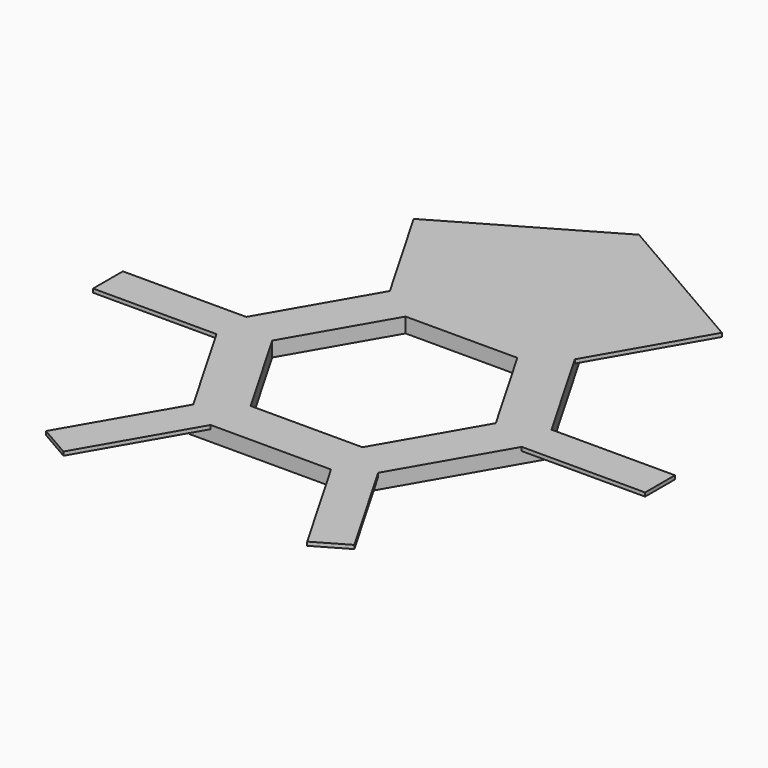
from build123d import *

# Parameters (mm, degrees)
F1_DEPTH = 152.4
F2_DEPTH = 457.2


# Not quite as in the source:
# - the program builds the solid bodies; features that only make, move or delete a surface that nothing else refers to are left out


with BuildPart() as f1:
    # F0 (on Top) → F1 (new body)
    with BuildSketch(Plane.XY):
        Polygon((6247.1608527394, 762), (6687.1017578619, 0), (6247.1608527394, -762), (11296.6448630235, -762), (11296.6448630235, 762), align=None)
        Polygon((6247.1608527394, -762), (6687.1017578619, 0), (6247.1608527394, 762), (3783.4917840535, 5029.2), (3343.550878931, 5791.2), (2463.669068686, 5791.2), (-2463.669068686, 5791.2), (-3343.550878931, 5791.2), (-3783.4917840535, 5029.2), (-6247.1608527394, 762), (-6687.1017578619, 0), (-6247.1608527394, -762), (-3783.4917840535, -5029.2), (-3343.550878931, -5791.2), (-2463.669068686, -5791.2), (2463.669068686, -5791.2), (3343.550878931, -5791.2), (3783.4917840535, -5029.2), align=None)
        Polygon((2287.692706637, 3962.4), (4575.3854132739, 0), (2287.692706637, -3962.4), (-2287.692706637, -3962.4), (-4575.3854132739, 0), (-2287.692706637, 3962.4), align=None, mode=Mode.SUBTRACT)
        Polygon((6308.2337891955, -9402.1814289093), (3783.4917840535, -5029.2), (3343.550878931, -5791.2), (2463.669068686, -5791.2), (4988.411073828, -10164.1814289093), align=None)
        Polygon((3343.550878931, 5791.2), (3783.4917840535, 5029.2), (6308.2337891955, 9402.1814289093), (4988.411073828, 10164.1814289093), (2463.669068686, 5791.2), align=None)
        Polygon((-2463.669068686, 5791.2), (2463.669068686, 5791.2), (4988.411073828, 10164.1814289093), (0, 13044.2419052124), (-4988.411073828, 10164.1814289093), align=None)
        Polygon((-4988.411073828, -10164.1814289093), (-2463.669068686, -5791.2), (-3343.550878931, -5791.2), (-3783.4917840535, -5029.2), (-6308.2337891955, -9402.1814289093), align=None)
        Polygon((-3343.550878931, 5791.2), (-2463.669068686, 5791.2), (-4988.411073828, 10164.1814289093), (-6308.2337891955, 9402.1814289093), (-3783.4917840535, 5029.2), align=None)
        Polygon((-11296.6448630235, -762), (-6247.1608527394, -762), (-6687.1017578619, 0), (-6247.1608527394, 762), (-11296.6448630235, 762), align=None)
    extrude(amount=F1_DEPTH)

    # F0 (on Top) → F2 (join)
    with BuildSketch(Plane.XY):
        Polygon((6247.1608527394, -762), (6687.1017578619, 0), (6247.1608527394, 762), (3783.4917840535, 5029.2), (3343.550878931, 5791.2), (2463.669068686, 5791.2), (-2463.669068686, 5791.2), (-3343.550878931, 5791.2), (-3783.4917840535, 5029.2), (-6247.1608527394, 762), (-6687.1017578619, 0), (-6247.1608527394, -762), (-3783.4917840535, -5029.2), (-3343.550878931, -5791.2), (-2463.669068686, -5791.2), (2463.669068686, -5791.2), (3343.550878931, -5791.2), (3783.4917840535, -5029.2), align=None)
        Polygon((2287.692706637, 3962.4), (4575.3854132739, 0), (2287.692706637, -3962.4), (-2287.692706637, -3962.4), (-4575.3854132739, 0), (-2287.692706637, 3962.4), align=None, mode=Mode.SUBTRACT)
    extrude(amount=-F2_DEPTH)


solid = f1.part
